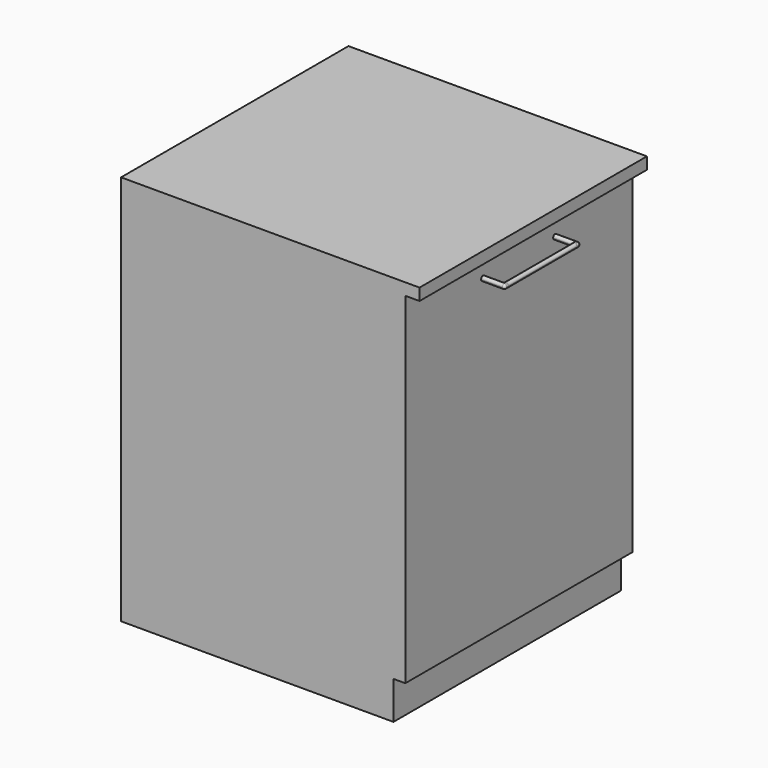
from build123d import *

# Parameters (mm, degrees)
F0_W          = 600
F0_H          = 600
F1_DEPTH      = 800
F2_W          = 600
F2_H          = 80
F3_DEPTH      = 25
F4_W          = 630
F4_H          = 600
F5_DEPTH      = 25
F7_DEPTH      = 50
F8_W          = 40
F8_H          = 180
F9_DEPTH      = 25
F10_T1_DEPTH  = 190
F10_T4_ANGLE  = 180
F10_T8_DEPTH  = 52.5
F10_S9_R      = 5
F10_T10_DEPTH = 28
F10_T14_DEPTH = 205
F10_S15_R     = 5
F10_T16_DEPTH = 104
F10_S17_R     = 5
F10_T18_DEPTH = 104
F10_T22_DEPTH = 52.5
F10_S23_R     = 5
F10_T24_DEPTH = 28
F10_T28_DEPTH = 52.5
F10_S29_R     = 5
F10_T30_DEPTH = 28
F10_T34_DEPTH = 205
F10_S35_R     = 5
F10_T36_DEPTH = 104
F10_S37_R     = 5
F10_T38_DEPTH = 104
F10_T42_DEPTH = 52.5
F10_S43_R     = 5
F10_T44_DEPTH = 28
F10_T46_ANGLE = 180


# Not quite as in the source:
# - a fillet or chamfer that OpenCascade refuses, or shapes differently, is made with other operations: its cross-section is extruded or revolved along the edge and cut away or added


with BuildPart() as f1:
    # F0 (on Top) → F1 (new body)
    with BuildSketch(Plane.XY):
        Rectangle(F0_W, F0_H)
    extrude(amount=F1_DEPTH)

    # F2 (on face) → F3 (cut)
    with BuildSketch(Plane.YZ.offset(300)):
        with Locations((0, 40)):
            Rectangle(F2_W, F2_H)
    extrude(amount=-F3_DEPTH, mode=Mode.SUBTRACT)

    # F4 (on face) → F5 (join)
    with BuildSketch(Plane.XY.offset(800)):
        with Locations((15, 0)):
            Rectangle(F4_W, F4_H)
    extrude(amount=F5_DEPTH)

    # F6 (on face) → F7 (join)
    with BuildSketch(Plane.YZ.offset(300)):
        with BuildLine():
            ThreePointArc((100, 749.2423057556), (98.5355339059, 752.7778396615), (95, 754.2423057556))
            Line((95, 754.2423057556), (-95, 754.2423057556))
            ThreePointArc((-95, 754.2423057556), (-98.5355339059, 752.7778396615), (-100, 749.2423057556))
            ThreePointArc((-100, 749.2423057556), (-98.5355339059, 745.7067718497), (-95, 744.2423057556))
            Line((-95, 744.2423057556), (95, 744.2423057556))
            ThreePointArc((95, 744.2423057556), (98.5355339059, 745.7067718497), (100, 749.2423057556))
        make_face()
    extrude(amount=F7_DEPTH)

    # F8 (on face) → F9 (cut)
    with BuildSketch(Plane(origin=(0, 0, 744.2423057556), x_dir=(1, 0, 0), z_dir=(0, 0, -1))):
        with Locations((320, 0)):
            Rectangle(F8_W, F8_H)
    extrude(amount=-F9_DEPTH, mode=Mode.SUBTRACT)

    # F10: fillet of radius 5 on 10 edges, made by hand

    # F10_s2 → F10_t1 (cut)
    with BuildSketch(Plane.XZ.offset(-95)):
        with BuildLine():
            ThreePointArc((345, 754.2423057556), (348.5355339059, 752.7778396615), (350, 749.2423057556))
            Line((350, 749.2423057556), (350, 754.2423057556))
            Line((350, 754.2423057556), (345, 754.2423057556))
        make_face()
        with BuildLine():
            ThreePointArc((345, 744.2423057556), (348.5355339059, 745.7067718497), (350, 749.2423057556))
            Line((350, 749.2423057556), (350, 744.2423057556))
            Line((350, 744.2423057556), (345, 744.2423057556))
        make_face()
    extrude(amount=F10_T1_DEPTH, mode=Mode.SUBTRACT)

    # F10_s3 → F10_t4 (revolve, cut)
    with BuildSketch(Plane.XZ.offset(-95)):
        with BuildLine():
            ThreePointArc((345, 754.2423057556), (348.5355339059, 752.7778396615), (350, 749.2423057556))
            Line((350, 749.2423057556), (350, 754.2423057556))
            Line((350, 754.2423057556), (345, 754.2423057556))
        make_face()
    revolve(axis=Axis((350, 95, 749.2423057556), (-1, 0, 0)), revolution_arc=F10_T4_ANGLE, mode=Mode.SUBTRACT)


with BuildPart() as f10_tool6:
    # F10_s7 → F10_t8 (new body)
    with BuildSketch(Plane.YZ.offset(300)):
        with BuildLine():
            ThreePointArc((95, 744.2423057556), (91.4644660941, 745.7067718497), (90, 749.2423057556))
            Line((90, 749.2423057556), (90, 744.2423057556))
            Line((90, 744.2423057556), (95, 744.2423057556))
        make_face()
    extrude(amount=F10_T8_DEPTH)

    # F10_s9 → F10_t10 (cut, symmetric)
    with BuildSketch(Plane.XZ.offset(-92.5)):
        with Locations((345, 749.2423057556)):
            Circle(F10_S9_R)
    extrude(amount=F10_T10_DEPTH, both=True, mode=Mode.SUBTRACT)


with BuildPart() as f1_1:
    add(f1.part)

    # F10_t5: cut F10_tool6
    add(f10_tool6.part, mode=Mode.SUBTRACT)


with BuildPart() as f10_tool12:
    # F10_s13 → F10_t14 (new body)
    with BuildSketch(Plane.XZ.offset(-102.5)):
        with BuildLine():
            ThreePointArc((345, 744.2423057556), (341.4644660941, 745.7067718497), (340, 749.2423057556))
            Line((340, 749.2423057556), (340, 744.2423057556))
            Line((340, 744.2423057556), (345, 744.2423057556))
        make_face()
    extrude(amount=F10_T14_DEPTH)

    # F10_s15 → F10_t16 (cut, symmetric)
    with BuildSketch(Plane.YZ.offset(342.5)):
        with Locations((-95, 749.2423057556)):
            Circle(F10_S15_R)
    extrude(amount=F10_T16_DEPTH, both=True, mode=Mode.SUBTRACT)

    # F10_s17 → F10_t18 (cut, symmetric)
    with BuildSketch(Plane.YZ.offset(342.5)):
        with Locations((95, 749.2423057556)):
            Circle(F10_S17_R)
    extrude(amount=F10_T18_DEPTH, both=True, mode=Mode.SUBTRACT)


with BuildPart() as f1_2:
    add(f1_1.part)

    # F10_t11: cut F10_tool12
    add(f10_tool12.part, mode=Mode.SUBTRACT)


with BuildPart() as f10_tool20:
    # F10_s21 → F10_t22 (new body)
    with BuildSketch(Plane.YZ.offset(352.5)):
        with BuildLine():
            ThreePointArc((-95, 744.2423057556), (-91.4644660941, 745.7067718497), (-90, 749.2423057556))
            Line((-90, 749.2423057556), (-90, 744.2423057556))
            Line((-90, 744.2423057556), (-95, 744.2423057556))
        make_face()
    extrude(amount=-F10_T22_DEPTH)

    # F10_s23 → F10_t24 (cut, symmetric)
    with BuildSketch(Plane.XZ.offset(92.5)):
        with Locations((345, 749.2423057556)):
            Circle(F10_S23_R)
    extrude(amount=F10_T24_DEPTH, both=True, mode=Mode.SUBTRACT)


with BuildPart() as f1_3:
    add(f1_2.part)

    # F10_t19: cut F10_tool20
    add(f10_tool20.part, mode=Mode.SUBTRACT)


with BuildPart() as f10_tool26:
    # F10_s27 → F10_t28 (new body)
    with BuildSketch(Plane.YZ.offset(300)):
        with BuildLine():
            ThreePointArc((95, 754.2423057556), (91.4644660941, 752.7778396615), (90, 749.2423057556))
            Line((90, 749.2423057556), (90, 754.2423057556))
            Line((90, 754.2423057556), (95, 754.2423057556))
        make_face()
    extrude(amount=F10_T28_DEPTH)

    # F10_s29 → F10_t30 (cut, symmetric)
    with BuildSketch(Plane.XZ.offset(-92.5)):
        with Locations((345, 749.2423057556)):
            Circle(F10_S29_R)
    extrude(amount=F10_T30_DEPTH, both=True, mode=Mode.SUBTRACT)


with BuildPart() as f1_4:
    add(f1_3.part)

    # F10_t25: cut F10_tool26
    add(f10_tool26.part, mode=Mode.SUBTRACT)


with BuildPart() as f10_tool32:
    # F10_s33 → F10_t34 (new body)
    with BuildSketch(Plane.XZ.offset(-102.5)):
        with BuildLine():
            ThreePointArc((345, 754.2423057556), (341.4644660941, 752.7778396615), (340, 749.2423057556))
            Line((340, 749.2423057556), (340, 754.2423057556))
            Line((340, 754.2423057556), (345, 754.2423057556))
        make_face()
    extrude(amount=F10_T34_DEPTH)

    # F10_s35 → F10_t36 (cut, symmetric)
    with BuildSketch(Plane.YZ.offset(342.5)):
        with Locations((95, 749.2423057556)):
            Circle(F10_S35_R)
    extrude(amount=F10_T36_DEPTH, both=True, mode=Mode.SUBTRACT)

    # F10_s37 → F10_t38 (cut, symmetric)
    with BuildSketch(Plane.YZ.offset(342.5)):
        with Locations((-95, 749.2423057556)):
            Circle(F10_S37_R)
    extrude(amount=F10_T38_DEPTH, both=True, mode=Mode.SUBTRACT)


with BuildPart() as f1_5:
    add(f1_4.part)

    # F10_t31: cut F10_tool32
    add(f10_tool32.part, mode=Mode.SUBTRACT)


with BuildPart() as f10_tool40:
    # F10_s41 → F10_t42 (new body)
    with BuildSketch(Plane.YZ.offset(352.5)):
        with BuildLine():
            ThreePointArc((-95, 754.2423057556), (-91.4644660941, 752.7778396615), (-90, 749.2423057556))
            Line((-90, 749.2423057556), (-90, 754.2423057556))
            Line((-90, 754.2423057556), (-95, 754.2423057556))
        make_face()
    extrude(amount=-F10_T42_DEPTH)

    # F10_s43 → F10_t44 (cut, symmetric)
    with BuildSketch(Plane.XZ.offset(92.5)):
        with Locations((345, 749.2423057556)):
            Circle(F10_S43_R)
    extrude(amount=F10_T44_DEPTH, both=True, mode=Mode.SUBTRACT)


with BuildPart() as f1_6:
    add(f1_5.part)

    # F10_t39: cut F10_tool40
    add(f10_tool40.part, mode=Mode.SUBTRACT)

    # F10_s45 → F10_t46 (revolve, cut)
    with BuildSketch(Plane.XZ.offset(95)):
        with BuildLine():
            ThreePointArc((345, 744.2423057556), (348.5355339059, 745.7067718497), (350, 749.2423057556))
            Line((350, 749.2423057556), (350, 744.2423057556))
            Line((350, 744.2423057556), (345, 744.2423057556))
        make_face()
    revolve(axis=Axis((350, -95, 749.2423057556), (-1, 0, 0)), revolution_arc=F10_T46_ANGLE, mode=Mode.SUBTRACT)


solid = f1_6.part
